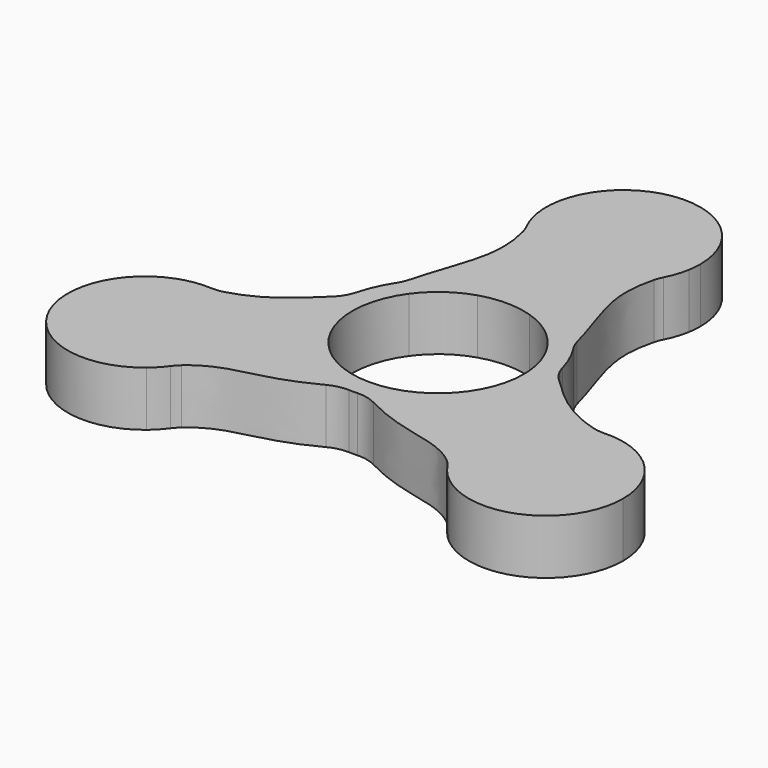
from build123d import *

# Parameters (mm, degrees)
F1_DEPTH = 7.1
F2_R     = 5


with BuildPart() as f1:
    # F0 (on Top) → F1 (new body)
    with BuildSketch(Plane.XY):
        with BuildLine():
            ThreePointArc((8.9370326257, 6.5832703003), (10.5454033148, 3.4647465892), (11.1, 0))
            ThreePointArc((11.1, 0), (-3.4287069831, -10.5571761577), (-8.9817961125, 6.5220655159))
            add(Edge.make_bspline(
                [(-8.9817961125, 6.5220655159), (-10.0885546906, 5.598589102), (-11.073678016, 4.6962067221), (-11.9818548247, 3.8269802204)],
                knots=[8.0142235912, 8.0142235912, 8.0142235912, 8.0142235912, 11.835160726, 11.835160726, 11.835160726, 11.835160726], degree=3))
            add(Edge.make_bspline(
                [(-11.9818548247, 3.8269802204), (-12.5324534616, 3.2999959124), (-13.0547695583, 2.7851984129), (-13.5587615762, 2.2852755894)],
                knots=[11.835160726, 11.835160726, 11.835160726, 11.835160726, 14.151673059, 14.151673059, 14.151673059, 14.151673059], degree=3))
            ThreePointArc((-13.5587615762, 2.2852755894), (-11.0674414121, -8.159303928), (-1.8268673691, -13.628098019))
            add(Edge.make_bspline(
                [(0, -12.5), (-0.6358071261, -12.9146274891), (-1.2439926916, -13.2890160563), (-1.8268673691, -13.628098019)],
                knots=[0, 0, 0, 0, 1.3161738098, 1.3161738098, 1.3161738098, 1.3161738098], degree=3))
            add(Edge.make_bspline(
                [(0, -12.5), (0.6364398741, -12.9150401216), (1.2469208398, -13.289088877), (1.8334533442, -13.6272135389)],
                knots=[0, 0, 0, 0, 1.317483651, 1.317483651, 1.317483651, 1.317483651], degree=3))
            ThreePointArc((1.8334533442, -13.6272135389), (10.3506638309, -9.0513125158), (13.75, 0))
            ThreePointArc((13.75, 0), (13.69932372, 1.1794191854), (13.5476684197, 2.3501447596))
            add(Edge.make_bspline(
                [(11.9733126897, 3.8777836857), (12.5230805512, 3.3555110401), (13.0444938727, 2.8454754224), (13.5476684197, 2.3501447596)],
                knots=[11.8509217323, 11.8509217323, 11.8509217323, 11.8509217323, 14.1735998792, 14.1735998792, 14.1735998792, 14.1735998792], degree=3))
            add(Edge.make_bspline(
                [(8.9370326257, 6.5832703003), (10.0594331527, 5.6550087301), (11.0558555016, 4.7493566284), (11.9733126897, 3.8777836857)],
                knots=[7.9748170878, 7.9748170878, 7.9748170878, 7.9748170878, 11.8509217323, 11.8509217323, 11.8509217323, 11.8509217323], degree=3))
        make_face()
        with BuildLine():
            ThreePointArc((3.3599585459, 10.5792569952), (6.4649806948, 9.02297205), (8.9370326257, 6.5832703003))
            add(Edge.make_bspline(
                [(8.9370326257, 6.5832703003), (10.0594331527, 5.6550087301), (11.0558555016, 4.7493566284), (11.9733126897, 3.8777836857)],
                knots=[7.9748170878, 7.9748170878, 7.9748170878, 7.9748170878, 11.8509217323, 11.8509217323, 11.8509217323, 11.8509217323], degree=3))
            add(Edge.make_bspline(
                [(11.0801114165, 8.1420900879), (11.4004506348, 6.8714368728), (11.7059070709, 5.4638269258), (11.9733126897, 3.8777836857)],
                knots=[22.6744965082, 22.6744965082, 22.6744965082, 22.6744965082, 25.9814012577, 25.9814012577, 25.9814012577, 25.9814012577], degree=3))
            ThreePointArc((11.0801114165, 8.1420900879), (3.98e-08, 13.75), (-11.0801113693, 8.142090152))
            add(Edge.make_bspline(
                [(-11.0801113693, 8.142090152), (-11.4038668249, 6.8578861908), (-11.7124203732, 5.4337887921), (-11.9818548247, 3.8269802204)],
                knots=[22.6744963996, 22.6744963996, 22.6744963996, 22.6744963996, 26.0166673605, 26.0166673605, 26.0166673605, 26.0166673605], degree=3))
            add(Edge.make_bspline(
                [(-8.9817961125, 6.5220655159), (-10.0885546906, 5.598589102), (-11.073678016, 4.6962067221), (-11.9818548247, 3.8269802204)],
                knots=[8.0142235912, 8.0142235912, 8.0142235912, 8.0142235912, 11.835160726, 11.835160726, 11.835160726, 11.835160726], degree=3))
            ThreePointArc((-8.9817961125, 6.5220655159), (-6.4912394293, 9.0040996591), (-3.3493267736, 10.5826277532))
            add(Edge.make_bspline(
                [(0, 12.5), (-1.2075190331, 11.8615533346), (-2.3195645537, 11.2212425381), (-3.3493267736, 10.5826277532)],
                knots=[0, 0, 0, 0, 2.5440235539, 2.5440235539, 2.5440235539, 2.5440235539], degree=3))
            add(Edge.make_bspline(
                [(0, 12.5), (1.2121818578, 11.8590879781), (2.3276857993, 11.2177467848), (3.3599585459, 10.5792569952)],
                knots=[0, 0, 0, 0, 2.5538472796, 2.5538472796, 2.5538472796, 2.5538472796], degree=3))
        make_face()
        with BuildLine():
            ThreePointArc((-3.3493267736, 10.5826277532), (0.005576661, 11.0999985991), (3.3599585459, 10.5792569952))
            add(Edge.make_bspline(
                [(0, 12.5), (1.2121818578, 11.8590879781), (2.3276857993, 11.2177467848), (3.3599585459, 10.5792569952)],
                knots=[0, 0, 0, 0, 2.5538472796, 2.5538472796, 2.5538472796, 2.5538472796], degree=3))
            add(Edge.make_bspline(
                [(0, 12.5), (-1.2075190331, 11.8615533346), (-2.3195645537, 11.2212425381), (-3.3493267736, 10.5826277532)],
                knots=[0, 0, 0, 0, 2.5440235539, 2.5440235539, 2.5440235539, 2.5440235539], degree=3))
        make_face()
        with BuildLine():
            add(Edge.make_bspline(
                [(11.0801114165, 8.1420900879), (11.4004506348, 6.8714368728), (11.7059070709, 5.4638269258), (11.9733126897, 3.8777836857)],
                knots=[22.6744965082, 22.6744965082, 22.6744965082, 22.6744965082, 25.9814012577, 25.9814012577, 25.9814012577, 25.9814012577], degree=3))
            add(Edge.make_bspline(
                [(11.9733126897, 3.8777836857), (12.5230805512, 3.3555110401), (13.0444938727, 2.8454754224), (13.5476684197, 2.3501447596)],
                knots=[11.8509217323, 11.8509217323, 11.8509217323, 11.8509217323, 14.1735998792, 14.1735998792, 14.1735998792, 14.1735998792], degree=3))
            ThreePointArc((13.5476684197, 2.3501447596), (12.6498435795, 5.3892446052), (11.0801114165, 8.1420900879))
        make_face()
        with BuildLine():
            add(Edge.make_bspline(
                [(-11.9818548247, 3.8269802204), (-12.5324534616, 3.2999959124), (-13.0547695583, 2.7851984129), (-13.5587615762, 2.2852755894)],
                knots=[11.835160726, 11.835160726, 11.835160726, 11.835160726, 14.151673059, 14.151673059, 14.151673059, 14.151673059], degree=3))
            add(Edge.make_bspline(
                [(-11.0801113693, 8.142090152), (-11.4038668249, 6.8578861908), (-11.7124203732, 5.4337887921), (-11.9818548247, 3.8269802204)],
                knots=[22.6744963996, 22.6744963996, 22.6744963996, 22.6744963996, 26.0166673605, 26.0166673605, 26.0166673605, 26.0166673605], degree=3))
            ThreePointArc((-11.0801113693, 8.142090152), (-12.6627044588, 5.3589565951), (-13.5587615762, 2.2852755894))
        make_face()
        with BuildLine():
            ThreePointArc((-11.0801113693, 8.142090152), (3.98e-08, 13.75), (11.0801114165, 8.1420900879))
            add(Edge.make_bspline(
                [(8.6546906258, 24.9903762446), (6.7470556094, 18.4077034644), (9.1763921895, 15.693357051), (11.0801114165, 8.1420900879)],
                knots=[3.0221473941, 3.0221473941, 3.0221473941, 3.0221473941, 22.6744965082, 22.6744965082, 22.6744965082, 22.6744965082], degree=3))
            ThreePointArc((8.6546906258, 24.9903762446), (-1.07e-08, 20), (-8.6546906366, 24.9903762631))
            add(Edge.make_bspline(
                [(-8.6546906366, 24.9903762631), (-6.74705547, 18.407703132), (-9.1763920992, 15.6933569666), (-11.0801113693, 8.142090152)],
                knots=[3.0221472191, 3.0221472191, 3.0221472191, 3.0221472191, 22.6744963996, 22.6744963996, 22.6744963996, 22.6744963996], degree=3))
        make_face()
        with BuildLine():
            add(Edge.make_bspline(
                [(13.5476684197, 2.3501447596), (17.0797943657, -1.1269196043), (19.7131873087, -3.879383298), (24.9469064988, -5.053586447)],
                knots=[14.1735998792, 14.1735998792, 14.1735998792, 14.1735998792, 30.4780647949, 30.4780647949, 30.4780647949, 30.4780647949], degree=3))
            ThreePointArc((13.5476684197, 2.3501447596), (13.69932372, 1.1794191854), (13.75, 0))
            ThreePointArc((13.75, 0), (10.3506638309, -9.0513125158), (1.8334533442, -13.6272135389))
            add(Edge.make_bspline(
                [(1.8334533442, -13.6272135389), (9.7028430683, -18.1637647449), (13.2612572959, -16.2336004445), (17.3642584266, -20.0750235677)],
                knots=[1.317483651, 1.317483651, 1.317483651, 1.317483651, 18.993899242, 18.993899242, 18.993899242, 18.993899242], degree=3))
            ThreePointArc((17.3642584266, -20.0750235677), (17.0536544097, -10.4936990731), (24.9469064988, -5.053586447))
        make_face()
        with BuildLine():
            ThreePointArc((-1.8268673691, -13.628098019), (-11.0674414121, -8.159303928), (-13.5587615762, 2.2852755894))
            add(Edge.make_bspline(
                [(-13.5587615762, 2.2852755894), (-17.0582662721, -1.1859743635), (-19.6743087226, -3.9400687723), (-24.7407002121, -5.0771855565)],
                knots=[14.151673059, 14.151673059, 14.151673059, 14.151673059, 30.2365424605, 30.2365424605, 30.2365424605, 30.2365424605], degree=3))
            ThreePointArc((-24.7407002121, -5.0771855565), (-18.484075545, -8.3818665401), (-15.9807621135, -15))
            ThreePointArc((-15.9807621135, -15), (-16.4077495602, -17.8909221113), (-17.6522482442, -20.5349667324))
            add(Edge.make_bspline(
                [(-1.8268673691, -13.628098019), (-9.9197965364, -18.3360848495), (-13.1333025427, -16.2376781384), (-17.6522482442, -20.5349667324)],
                knots=[1.3161738098, 1.3161738098, 1.3161738098, 1.3161738098, 19.5906019581, 19.5906019581, 19.5906019581, 19.5906019581], degree=3))
        make_face()
        with BuildLine():
            add(Edge.make_bspline(
                [(9.8601329718, 28.3333333333), (9.3439672033, 27.1064290641), (8.9480476266, 26.0026627287), (8.6546906258, 24.9903762446)],
                knots=[0, 0, 0, 0, 3.0221473941, 3.0221473941, 3.0221473941, 3.0221473941], degree=3))
            ThreePointArc((8.6546906258, 24.9903762446), (9.4070991138, 26.607878796), (9.8601329718, 28.3333333333))
        make_face()
        with BuildLine():
            ThreePointArc((-8.6546906366, 24.9903762631), (-1.07e-08, 20), (8.6546906258, 24.9903762446))
            add(Edge.make_bspline(
                [(9.8601329718, 28.3333333333), (9.3439672033, 27.1064290641), (8.9480476266, 26.0026627287), (8.6546906258, 24.9903762446)],
                knots=[0, 0, 0, 0, 3.0221473941, 3.0221473941, 3.0221473941, 3.0221473941], degree=3))
            ThreePointArc((9.8601329718, 28.3333333333), (9.9649718945, 29.1637373972), (10, 30))
            ThreePointArc((10, 30), (-0.8362626028, 39.9649718945), (-9.8601329718, 28.3333333333))
            add(Edge.make_bspline(
                [(-9.8601329718, 28.3333333333), (-9.3439672164, 27.1064290695), (-8.9480476424, 26.0026627391), (-8.6546906366, 24.9903762631)],
                knots=[0, 0, 0, 0, 3.0221472191, 3.0221472191, 3.0221472191, 3.0221472191], degree=3))
        make_face()
        with BuildLine():
            add(Edge.make_bspline(
                [(24.9469064988, -5.053586447), (26.2690167444, -5.3502064904), (27.7570636508, -5.5461117543), (29.4674529265, -5.6275410284)],
                knots=[30.4780647949, 30.4780647949, 30.4780647949, 30.4780647949, 34.5967993564, 34.5967993564, 34.5967993564, 34.5967993564], degree=3))
            ThreePointArc((24.9469064988, -5.053586447), (17.0536544097, -10.4936990731), (17.3642584266, -20.0750235677))
            add(Edge.make_bspline(
                [(17.3642584266, -20.0750235677), (18.0862629744, -20.7509982693), (18.8251308695, -21.6056924424), (19.6073199546, -22.705792305)],
                knots=[18.993899242, 18.993899242, 18.993899242, 18.993899242, 22.104415676, 22.104415676, 22.104415676, 22.104415676], degree=3))
            ThreePointArc((19.6073199546, -22.705792305), (30.2390234026, -24.0480501101), (35.9807621135, -15))
            ThreePointArc((35.9807621135, -15), (34.1925496208, -9.2932893945), (29.4674529265, -5.6275410284))
        make_face()
        with BuildLine():
            ThreePointArc((29.4674529265, -5.6275410284), (27.2403081003, -5.0796399306), (24.9469064988, -5.053586447))
            add(Edge.make_bspline(
                [(24.9469064988, -5.053586447), (26.2690167444, -5.3502064904), (27.7570636508, -5.5461117543), (29.4674529265, -5.6275410284)],
                knots=[30.4780647949, 30.4780647949, 30.4780647949, 30.4780647949, 34.5967993564, 34.5967993564, 34.5967993564, 34.5967993564], degree=3))
        make_face()
        with BuildLine():
            ThreePointArc((-9.8601329718, 28.3333333333), (-9.4070991175, 26.6078788061), (-8.6546906366, 24.9903762631))
            add(Edge.make_bspline(
                [(-9.8601329718, 28.3333333333), (-9.3439672164, 27.1064290695), (-8.9480476424, 26.0026627391), (-8.6546906366, 24.9903762631)],
                knots=[0, 0, 0, 0, 3.0221472191, 3.0221472191, 3.0221472191, 3.0221472191], degree=3))
        make_face()
        with BuildLine():
            add(Edge.make_bspline(
                [(-24.7407002121, -5.0771855565), (-26.1140883248, -5.3854330887), (-27.6675363474, -5.5748596526), (-29.4674529265, -5.6275410284)],
                knots=[30.2365424605, 30.2365424605, 30.2365424605, 30.2365424605, 34.5967993564, 34.5967993564, 34.5967993564, 34.5967993564], degree=3))
            ThreePointArc((-24.7407002121, -5.0771855565), (-27.1372906056, -5.0671030486), (-29.4674529265, -5.6275410284))
        make_face()
        with BuildLine():
            ThreePointArc((-15.9807621135, -15), (-18.484075545, -8.3818665401), (-24.7407002121, -5.0771855565))
            add(Edge.make_bspline(
                [(-24.7407002121, -5.0771855565), (-26.1140883248, -5.3854330887), (-27.6675363474, -5.5748596526), (-29.4674529265, -5.6275410284)],
                knots=[30.2365424605, 30.2365424605, 30.2365424605, 30.2365424605, 34.5967993564, 34.5967993564, 34.5967993564, 34.5967993564], degree=3))
            ThreePointArc((-29.4674529265, -5.6275410284), (-34.6410161514, -20), (-19.6073199546, -22.705792305))
            add(Edge.make_bspline(
                [(-17.6522482442, -20.5349667324), (-18.2738703055, -21.1260978435), (-18.9201945539, -21.8382515209), (-19.6073199546, -22.705792305)],
                knots=[19.5906019581, 19.5906019581, 19.5906019581, 19.5906019581, 22.104415676, 22.104415676, 22.104415676, 22.104415676], degree=3))
            ThreePointArc((-17.6522482442, -20.5349667324), (-16.4077495602, -17.8909221113), (-15.9807621135, -15))
        make_face()
        with BuildLine():
            add(Edge.make_bspline(
                [(0, -12.5), (-0.6358071261, -12.9146274891), (-1.2439926916, -13.2890160563), (-1.8268673691, -13.628098019)],
                knots=[0, 0, 0, 0, 1.3161738098, 1.3161738098, 1.3161738098, 1.3161738098], degree=3))
            ThreePointArc((-1.8268673691, -13.628098019), (0.0033225507, -13.7499995986), (1.8334533442, -13.6272135389))
            add(Edge.make_bspline(
                [(0, -12.5), (0.6364398741, -12.9150401216), (1.2469208398, -13.289088877), (1.8334533442, -13.6272135389)],
                knots=[0, 0, 0, 0, 1.317483651, 1.317483651, 1.317483651, 1.317483651], degree=3))
        make_face()
        with BuildLine():
            add(Edge.make_bspline(
                [(17.3642584266, -20.0750235677), (18.0862629744, -20.7509982693), (18.8251308695, -21.6056924424), (19.6073199546, -22.705792305)],
                knots=[18.993899242, 18.993899242, 18.993899242, 18.993899242, 22.104415676, 22.104415676, 22.104415676, 22.104415676], degree=3))
            ThreePointArc((17.3642584266, -20.0750235677), (18.3712381368, -21.4880771302), (19.6073199546, -22.705792305))
        make_face()
        with BuildLine():
            ThreePointArc((-19.6073199546, -22.705792305), (-18.5500825564, -21.6921596902), (-17.6522482442, -20.5349667324))
            add(Edge.make_bspline(
                [(-17.6522482442, -20.5349667324), (-18.2738703055, -21.1260978435), (-18.9201945539, -21.8382515209), (-19.6073199546, -22.705792305)],
                knots=[19.5906019581, 19.5906019581, 19.5906019581, 19.5906019581, 22.104415676, 22.104415676, 22.104415676, 22.104415676], degree=3))
        make_face()
    extrude(amount=F1_DEPTH)

    # F2
    f2_edges = [f1.edges().sort_by_distance(p)[0] for p in [
        (-17.652248, -20.534967, 3.55),
        (-24.7407, -5.077186, 3.55),
        (24.946906, -5.053586, 3.55),
        (17.364258, -20.075024, 3.55),
        (8.654691, 24.990376, 3.55),
        (-8.654691, 24.990376, 3.55),
        (-11.080111, 8.14209, 3.55),
        (-13.558762, 2.285276, 3.55),
        (11.080111, 8.14209, 3.55),
        (13.547668, 2.350145, 3.55),
        (1.833453, -13.627214, 3.55),
        (-1.826867, -13.628098, 3.55),
    ]]
    fillet(f2_edges, radius=F2_R)


solid = f1.part
